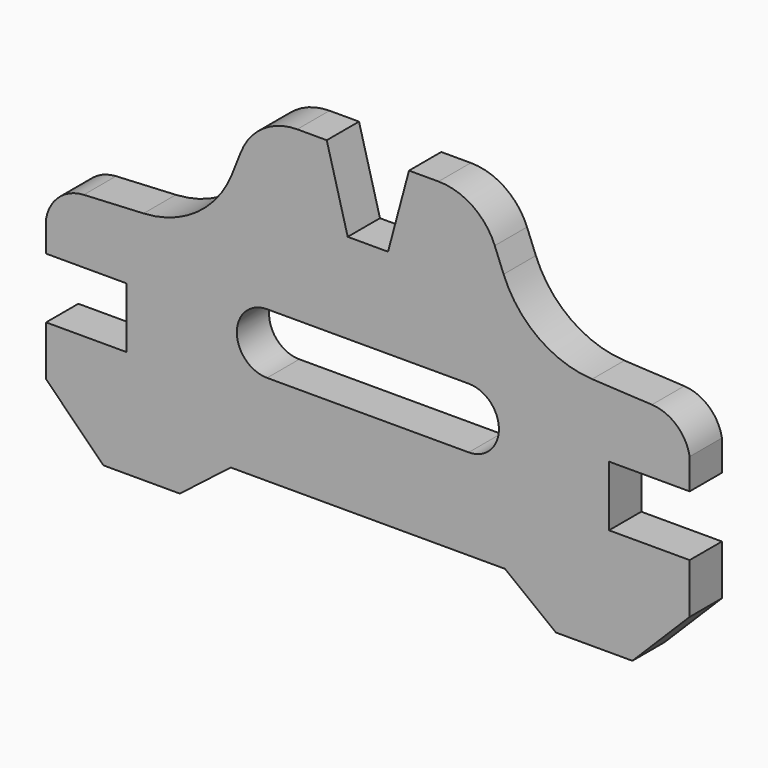
from build123d import *

# Parameters (mm, degrees)
F1_DEPTH     = 12.7
F2_T1_DEPTH  = 105.45546201
F2_T6_DEPTH  = 85.6153780659
F2_T11_DEPTH = 85.6153780659


# Not quite as in the source:
# - a fillet or chamfer that OpenCascade refuses, or shapes differently, is made with other operations: its cross-section is extruded or revolved along the edge and cut away or added


with BuildPart() as f1:
    # F0 (on Front) → F1 (new body)
    with BuildSketch(Plane.XZ):
        with BuildLine():
            Line((6.35, 54.2438933111), (-6.35, 54.2438933111))
            Line((-6.35, 54.2438933111), (-12.9517322031, 78.8818933111))
            Line((-12.9517322031, 78.8818933111), (-22.2531325433, 78.8818933111))
            ThreePointArc((-22.2531325433, 78.8818933111), (-32.9570059401, 75.5903702142), (-39.961976816, 66.8532417945))
            Line((-39.961976816, 66.8532417945), (-42.7458589128, 59.8318933111))
            ThreePointArc((-42.7458589128, 59.8318933111), (-53.7566077671, 45.7336602674), (-70.6412160864, 39.8254653493))
            Line((-70.6412160864, 39.8254653493), (-89.4780809568, 38.8634540506))
            ThreePointArc((-89.4780809568, 38.8634540506), (-97.258039529, 35.6807034492), (-101.346, 28.3358933111))
            Line((-101.346, 28.3358933111), (-101.346, 18.6838933111))
            Line((-101.346, 18.6838933111), (-75.946, 18.6838933111))
            Line((-75.946, 18.6838933111), (-75.946, -0.3661066889))
            Line((-75.946, -0.3661066889), (-101.346, -0.3661066889))
            Line((-101.346, -0.3661066889), (-101.346, -34.1481066889))
            Line((-101.346, -34.1481066889), (-45.212, -34.1481066889))
            Line((-45.212, -34.1481066889), (-42.0329745032, -21.7021066889))
            Line((-42.0329745032, -21.7021066889), (0, -21.7021066889))
            Line((0, -21.7021066889), (42.0329745032, -21.7021066889))
            Line((42.0329745032, -21.7021066889), (45.212, -34.1481066889))
            Line((45.212, -34.1481066889), (101.346, -34.1481066889))
            Line((101.346, -34.1481066889), (101.346, -0.3661066889))
            Line((101.346, -0.3661066889), (75.946, -0.3661066889))
            Line((75.946, -0.3661066889), (75.946, 18.6838933111))
            Line((75.946, 18.6838933111), (101.346, 18.6838933111))
            Line((101.346, 18.6838933111), (101.346, 28.3358933111))
            ThreePointArc((101.346, 28.3358933111), (97.258039529, 35.6807034492), (89.4780809568, 38.8634540506))
            Line((89.4780809568, 38.8634540506), (70.6412160864, 39.8254653493))
            ThreePointArc((70.6412160864, 39.8254653493), (53.7566077671, 45.7336602674), (42.7458589128, 59.8318933111))
            Line((42.7458589128, 59.8318933111), (39.961976816, 66.8532417945))
            ThreePointArc((39.961976816, 66.8532417945), (32.9570059401, 75.5903702142), (22.2531325433, 78.8818933111))
            Line((22.2531325433, 78.8818933111), (12.9517322031, 78.8818933111))
            Line((12.9517322031, 78.8818933111), (6.35, 54.2438933111))
        make_face()
        with BuildLine():
            ThreePointArc((-31.75, 6.8728933111), (-41.275, 16.3978933111), (-31.75, 25.9228933111))
            Line((-31.75, 25.9228933111), (31.75, 25.9228933111))
            ThreePointArc((31.75, 25.9228933111), (41.275, 16.3978933111), (31.75, 6.8728933111))
            Line((31.75, 6.8728933111), (-31.75, 6.8728933111))
        make_face(mode=Mode.SUBTRACT)
    extrude(amount=F1_DEPTH)

    # F2: chamfer of 18.034 on 4 edges, made by hand

    # F2_s2 → F2_t1 (cut)
    with BuildSketch(Plane.XZ.offset(-46.377731005)):
        Polygon((-101.346, -16.1141066889), (-83.312, -34.1481066889), (-101.346, -34.1481066889), align=None)
        Polygon((101.346, -16.1141066889), (83.312, -34.1481066889), (101.346, -34.1481066889), align=None)
    extrude(amount=F2_T1_DEPTH, mode=Mode.SUBTRACT)


with BuildPart() as f2_tool4:
    # F2_s5 → F2_t6 (new body)
    with BuildSketch(Plane.XZ.offset(-36.4576890329)):
        Polygon((-41.7456345338, -20.5771602982), (-59.218651116, -34.1481066889), (-45.212, -34.1481066889), align=None)
    extrude(amount=F2_T6_DEPTH)

    split(bisect_by=Plane.XY.offset(-21.7021066889), keep=Keep.BOTTOM)


with BuildPart() as f1_1:
    add(f1.part)

    # F2_t3: cut F2_tool4
    add(f2_tool4.part, mode=Mode.SUBTRACT)


with BuildPart() as f2_tool9:
    # F2_s10 → F2_t11 (new body)
    with BuildSketch(Plane.XZ.offset(-36.4576890329)):
        Polygon((59.218651116, -34.1481066889), (41.7456345338, -20.5771602982), (45.212, -34.1481066889), align=None)
    extrude(amount=F2_T11_DEPTH)

    split(bisect_by=Plane.XY.offset(-21.7021066889), keep=Keep.BOTTOM)


with BuildPart() as f1_2:
    add(f1_1.part)

    # F2_t8: cut F2_tool9
    add(f2_tool9.part, mode=Mode.SUBTRACT)


solid = f1_2.part
